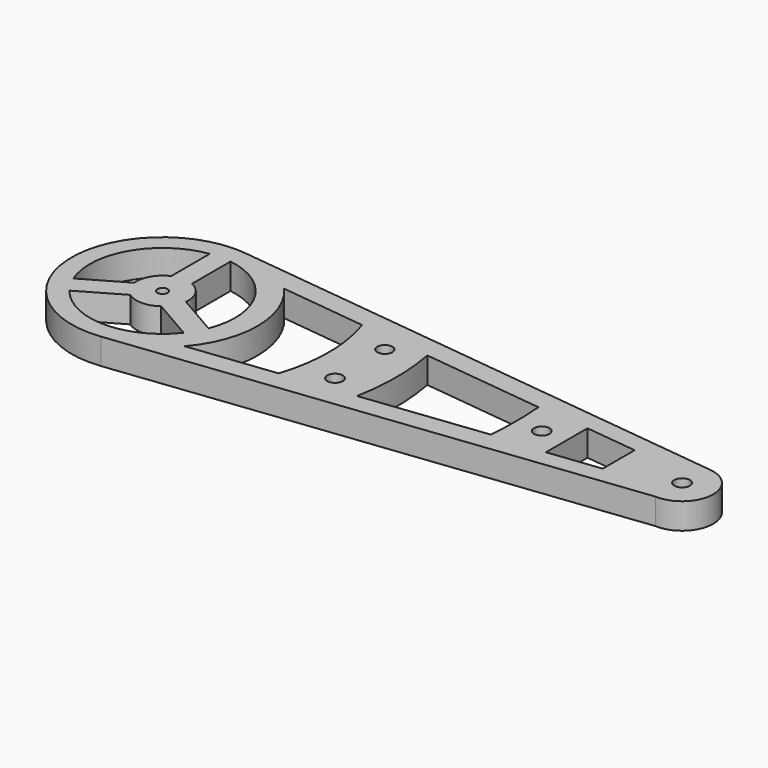
from build123d import *

# Parameters (mm, degrees)
F0_R     = 1.5
F1_DEPTH = 5
F2_W     = 5
F2_H     = 5
F2_H_2   = 4.5
F2_R     = 3.5
F3_DEPTH = 3
F4_R     = 1.5
F4_R_2   = 1.4524317573
F5_DEPTH = 25
F6_R     = 3
F7_DEPTH = 7
F8_SIZE  = 1.99999
F9_DEPTH = 25


# Not quite as in the source:
# - a fillet or chamfer is up to 0.001 mm smaller than in the source, because OpenCascade refuses the exact size


with BuildPart() as f1:
    # F0 (on Top) → F1 (new body)
    with BuildSketch(Plane.XY):
        with BuildLine():
            Line((100.4699678509, 5.9815658668), (2.0132142916, 17.3838133968))
            ThreePointArc((2.0132142916, 17.3838133968), (-17.4999985209, -0.0071949455), (2.027507963, -17.3821520952))
            Line((2.027507963, -17.3821520952), (99.6811939192, -5.991524237))
            ThreePointArc((99.6811939192, -5.991524237), (105.987022142, -0.394418396), (100.4699678509, 5.9815658668))
        make_face()
        with BuildLine():
            Line((-11, -8.6602540378), (-2.9686269666, -4.023338655))
            ThreePointArc((-2.9686269666, -4.023338655), (0, -5), (2.9686269666, -4.023338655))
            Line((2.9686269666, -4.023338655), (11, -8.6602540378))
            ThreePointArc((11, -8.6602540378), (0, -14), (-11, -8.6602540378))
        make_face(mode=Mode.SUBTRACT)
        with BuildLine():
            ThreePointArc((-13, -5.1961524227), (-12.124355653, 7), (-2, 13.8564064606))
            Line((-2, 13.8564064606), (-2, 4.582575695))
            ThreePointArc((-2, 4.582575695), (-4.3301270189, 2.5), (-4.9686269666, -0.5592370399))
            Line((-4.9686269666, -0.5592370399), (-13, -5.1961524227))
        make_face(mode=Mode.SUBTRACT)
        Circle(F0_R, mode=Mode.SUBTRACT)
        with BuildLine():
            Line((2, 4.582575695), (2, 13.8564064606))
            ThreePointArc((2, 13.8564064606), (12.124355653, 7), (13, -5.1961524227))
            Line((13, -5.1961524227), (4.9686269666, -0.5592370399))
            ThreePointArc((4.9686269666, -0.5592370399), (4.3301270189, 2.5), (2, 4.582575695))
        make_face(mode=Mode.SUBTRACT)
        with BuildLine():
            Line((30.3816278502, -10.0477205958), (13.8356347618, -11.9776963869))
            ThreePointArc((13.8356347618, -11.9776963869), (18.2999984533, 0.0075238573), (13.8257810711, 11.9890690954))
            Line((13.8257810711, 11.9890690954), (30.3733555452, 10.0726993863))
            ThreePointArc((30.3733555452, 10.0726993863), (31.9999972954, 0.0131564719), (30.3816278502, -10.0477205958))
        make_face(mode=Mode.SUBTRACT)
        with BuildLine():
            Line((67.7617245486, -5.6875905441), (44.2022623135, -8.435639061))
            ThreePointArc((44.2022623135, -8.435639061), (44.9999961967, 0.0185012885), (44.1953109176, 8.4719828198))
            Line((44.1953109176, 8.4719828198), (67.7570248516, 5.743307693))
            ThreePointArc((67.7570248516, 5.743307693), (67.9999942528, 0.0279575027), (67.7617245486, -5.6875905441))
        make_face(mode=Mode.SUBTRACT)
        Polygon((77.8001793809, -5), (77.8001793809, 5), (87.8001793809, 3.8419029556), (87.8001793809, -3.8335690817), align=None, mode=Mode.SUBTRACT)
        with Locations((100, 0)):
            Circle(F0_R, mode=Mode.SUBTRACT)
    extrude(amount=F1_DEPTH)

    # F2 (on face) → F3 (cut)
    with BuildSketch(Plane(origin=(0, 0, 0), x_dir=(1, 0, 0), z_dir=(0, 0, -1))):
        with Locations((38, 6)):
            Rectangle(F2_W, F2_H)
        with Locations((73, 0)):
            Rectangle(F2_W, F2_H_2)
        with Locations((38, -6)):
            Rectangle(F2_W, F2_H)
        with Locations((100, 0)):
            Circle(F2_R)
    extrude(amount=-F3_DEPTH, mode=Mode.SUBTRACT)

    # F4 (on face) → F5 (cut)
    with BuildSketch(Plane.XY.offset(5)):
        with Locations((38, -6)):
            Circle(F4_R)
        with Locations((73, 0)):
            Circle(F4_R)
        with Locations((38, 6)):
            Circle(F4_R_2)
    extrude(amount=-F5_DEPTH, mode=Mode.SUBTRACT)

    # F6 (on face) → F7 (join)
    with BuildSketch(Plane.XY.offset(5)):
        Circle(F6_R)
    extrude(amount=-F7_DEPTH)

    # F8 (size 2 in the source; OpenCascade refuses exactly that, so slightly less here)
    f8_edges = [f1.edges().sort_by_distance(p)[0] for p in [
        (-3, 0, -2),
    ]]
    chamfer(f8_edges, length=F8_SIZE)

    # F9 (cut): a face of the model
    f9_faces = [f1.faces().sort_by_distance(p)[0] for p in [
        (0, 0, -2),
    ]]
    extrude(f9_faces, amount=-F9_DEPTH, mode=Mode.SUBTRACT)


solid = f1.part
